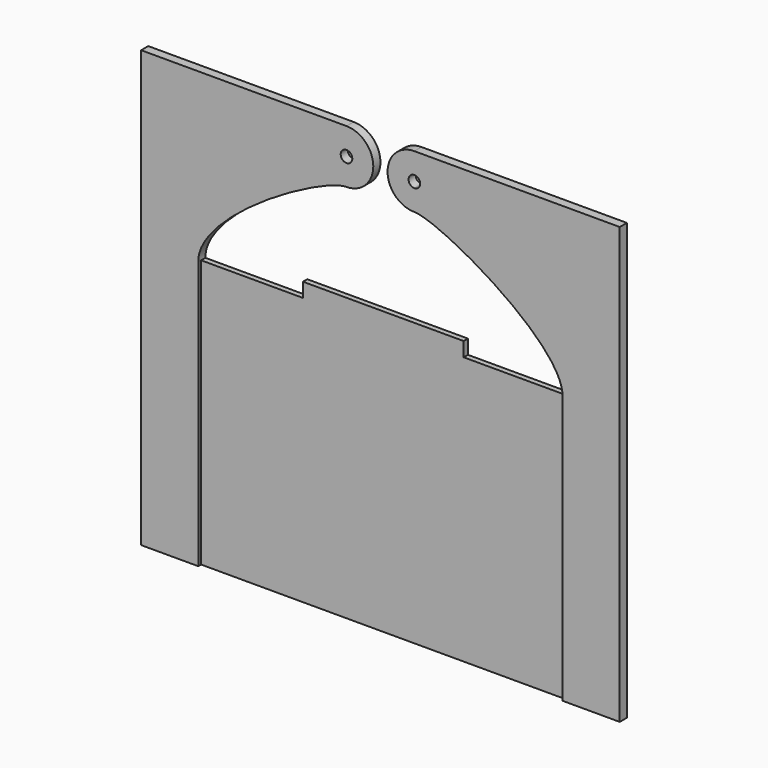
from build123d import *

# Parameters (mm, degrees)
F1_DEPTH = 3
F0_R     = 3.25
F2_DEPTH = 5
F0_W     = 32
F0_H     = 150


# Not quite as in the source:
# - a feature names something its author has since deleted; it is built from what else it names


with BuildPart() as f1:
    # F0 (on Front) → F1 (new body)
    with BuildSketch(Plane.XZ):
        Polygon((-45, 83), (-45, 75), (0, 75), (45, 75), (45, 83), align=None)
        Polygon((-45, 75), (-102, 75), (-102, -75), (102, -75), (102, 75), (45, 75), (0, 75), align=None)
    extrude(amount=F1_DEPTH)


with BuildPart() as f2:
    # F0 (on Front) → F2 (new body)
    with BuildSketch(Plane.XZ):
        Polygon((-104, 75), (-134, 75), (-134, -75), (-102, -75), (-102, 75), align=None)
        with BuildLine():
            Line((-134, 168.9787209958), (-134, 75))
            Line((-134, 75), (-104, 75))
            Line((-104, 75), (-102, 75))
            add(Edge.make_bspline(
                [(-19, 138.9787209958), (-33.9978419072, 138.7242841167), (-102.5319148936, 99.9943406904), (-102, 75)],
                knots=[0, 0, 0, 0, 104.7963584303, 104.7963584303, 104.7963584303, 104.7963584303], degree=3))
            ThreePointArc((-19, 138.9787209958), (-4, 153.9787209958), (-19, 168.9787209958))
            Line((-19, 168.9787209958), (-104, 168.9787209958))
            Line((-104, 168.9787209958), (-134, 168.9787209958))
        make_face()
        with Locations((-19, 153.9787209958)):
            Circle(F0_R, mode=Mode.SUBTRACT)
    extrude(amount=F2_DEPTH)


with BuildPart() as f2b:
    # F0 (on Front) → F2, piece 2 (new body)
    with BuildSketch(Plane.XZ):
        with Locations((118, 0)):
            Rectangle(F0_W, F0_H)
        Polygon((104, 168.9787209958), (102, 75), (134, 75), (134, 168.9787209958), align=None)
        with BuildLine():
            add(Edge.make_bspline(
                [(19, 138.9787209958), (33.9978419072, 138.7242841167), (102.5319148936, 99.9943406904), (102, 75)],
                knots=[0, 0, 0, 0, 104.7963584303, 104.7963584303, 104.7963584303, 104.7963584303], degree=3))
            Line((102, 75), (104, 168.9787209958))
            Line((104, 168.9787209958), (19, 168.9787209958))
            Line((19, 168.9787209958), (19, 157.2287209958))
            ThreePointArc((19, 157.2287209958), (21.2980970389, 156.2768180346), (22.25, 153.9787209958))
            ThreePointArc((22.25, 153.9787209958), (21.2980970389, 151.6806239569), (19, 150.7287209958))
            Line((19, 150.7287209958), (19, 138.9787209958))
        make_face()
        with BuildLine():
            ThreePointArc((19, 168.9787209958), (4, 153.9787209958), (19, 138.9787209958))
            Line((19, 138.9787209958), (19, 150.7287209958))
            ThreePointArc((19, 150.7287209958), (15.75, 153.9787209958), (19, 157.2287209958))
            Line((19, 157.2287209958), (19, 168.9787209958))
        make_face()
    extrude(amount=F2_DEPTH)


solid = Compound([f1.part, f2.part, f2b.part])
